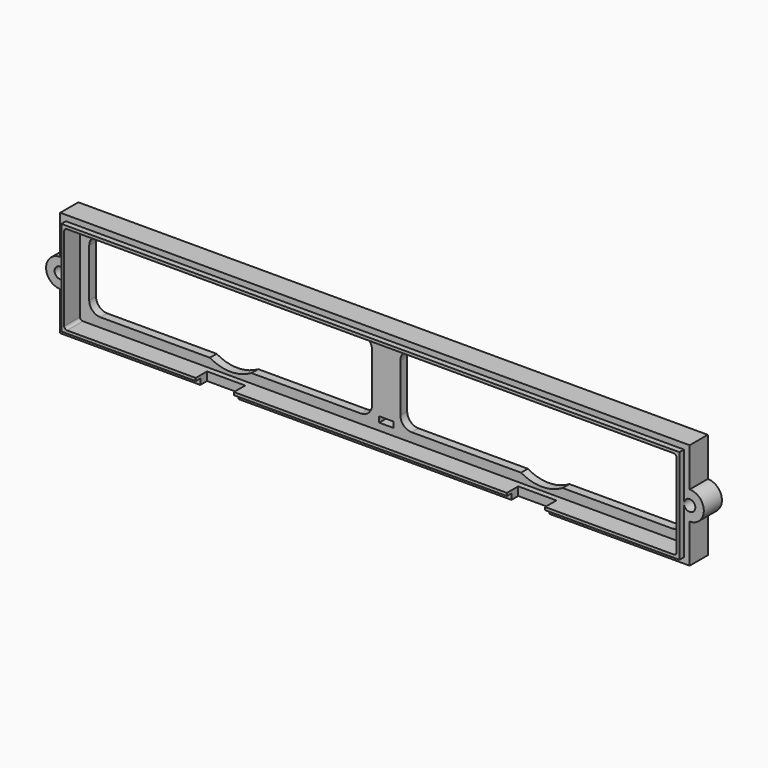
from build123d import *

# Parameters (mm, degrees)
F0_W        = 5
F0_H        = 2
F1_DEPTH    = 3
F2_R        = 2
F3_DEPTH    = 5
F4_W        = 218.5
F4_H        = 33.5
F5_DEPTH    = 2
F6_W        = 13.5
F6_H        = 5
F7_DEPTH    = 25
F8_T1_DEPTH = 5


# Not quite as in the source:
# - a fillet or chamfer that OpenCascade refuses, or shapes differently, is made with other operations: its cross-section is extruded or revolved along the edge and cut away or added
# - a feature names something its author has since deleted; it is built from what else it names


with BuildPart() as f1:
    # F0 (on Front) → F1 (new body)
    with BuildSketch(Plane.XZ):
        Polygon((111.25, 5), (111.25, 18.75), (-111.25, 18.75), (-111.25, 5), (-111.25, -5), (-111.25, -18.75), (111.25, -18.75), (111.25, -5), align=None)
        with Locations((0, -12.25)):
            Rectangle(F0_W, F0_H, mode=Mode.SUBTRACT)
        with BuildLine():
            Line((-47.6515307717, 12.5), (-9, 12.5))
            ThreePointArc((-9, 12.5), (-6.1715728753, 11.3284271247), (-5, 8.5))
            Line((-5, 8.5), (-5, -8.5))
            ThreePointArc((-5, -8.5), (-6.1715728753, -11.3284271247), (-9, -12.5))
            Line((-9, -12.5), (-47.6515307717, -12.5))
            ThreePointArc((-47.6515307717, -12.5), (-55, -14.5), (-62.3484692283, -12.5))
            Line((-62.3484692284, -12.5), (-101, -12.5))
            ThreePointArc((-101, -12.5), (-103.8284271247, -11.3284271247), (-105, -8.5))
            Line((-105, -8.5), (-105, 8.5))
            ThreePointArc((-105, 8.5), (-103.8284271247, 11.3284271247), (-101, 12.5))
            Line((-101, 12.5), (-62.3484692284, 12.5))
            ThreePointArc((-62.3484692283, 12.5), (-55, 14.5), (-47.6515307717, 12.5))
        make_face(mode=Mode.SUBTRACT)
        with BuildLine():
            Line((62.3484692283, 12.5), (101, 12.5))
            ThreePointArc((101, 12.5), (103.8284271247, 11.3284271247), (105, 8.5))
            Line((105, 8.5), (105, -8.5))
            ThreePointArc((105, -8.5), (103.8284271247, -11.3284271247), (101, -12.5))
            Line((101, -12.5), (62.3484692283, -12.5))
            ThreePointArc((62.3484692283, -12.5), (55, -14.5), (47.6515307717, -12.5))
            Line((47.6515307716, -12.5), (9, -12.5))
            ThreePointArc((9, -12.5), (6.1715728753, -11.3284271247), (5, -8.5))
            Line((5, -8.5), (5, 8.5))
            ThreePointArc((5, 8.5), (6.1715728753, 11.3284271247), (9, 12.5))
            Line((9, 12.5), (47.6515307716, 12.5))
            ThreePointArc((47.6515307717, 12.5), (55, 14.5), (62.3484692283, 12.5))
        make_face(mode=Mode.SUBTRACT)
        with Locations((0, 12.25)):
            Rectangle(F0_W, F0_H, mode=Mode.SUBTRACT)
        with BuildLine():
            ThreePointArc((111.25, -5), (116.25, 0), (111.25, 5))
            Line((111.25, 5), (111.25, -5))
        make_face()
        with BuildLine():
            Line((-111.25, -5), (-111.25, 5))
            ThreePointArc((-111.25, 5), (-116.25, 0), (-111.25, -5))
        make_face()
    extrude(amount=F1_DEPTH)

    # F2 (on face) → F3 (join)
    with BuildSketch(Plane.XZ.offset(3)):
        with BuildLine():
            ThreePointArc((111.25, -5), (116.25, 0), (111.25, 5))
            Line((111.25, 5), (111.25, 18.75))
            Line((111.25, 18.75), (-111.25, 18.75))
            Line((-111.25, 18.75), (-111.25, 5))
            ThreePointArc((-111.25, 5), (-116.25, 0), (-111.25, -5))
            Line((-111.25, -5), (-111.25, -18.75))
            Line((-111.25, -18.75), (111.25, -18.75))
            Line((111.25, -18.75), (111.25, -5))
        make_face()
        with Locations((-111.25, 0)):
            Circle(F2_R, mode=Mode.SUBTRACT)
        with BuildLine():
            Line((-107.25, 15.75), (107.25, 15.75))
            ThreePointArc((107.25, 15.75), (107.9571067812, 15.4571067812), (108.25, 14.75))
            Line((108.25, 14.75), (108.25, -14.75))
            ThreePointArc((108.25, -14.75), (107.9571067812, -15.4571067812), (107.25, -15.75))
            Line((107.25, -15.75), (-107.25, -15.75))
            ThreePointArc((-107.25, -15.75), (-107.9571067812, -15.4571067812), (-108.25, -14.75))
            Line((-108.25, -14.75), (-108.25, 14.75))
            ThreePointArc((-108.25, 14.75), (-107.9571067812, 15.4571067812), (-107.25, 15.75))
        make_face(mode=Mode.SUBTRACT)
        with Locations((111.25, 0)):
            Circle(F2_R, mode=Mode.SUBTRACT)
    extrude(amount=F3_DEPTH)

    # F4 (on face) → F5 (join)
    with BuildSketch(Plane.XZ.offset(8)):
        Rectangle(F4_W, F4_H)
        with BuildLine():
            ThreePointArc((-108.25, 14.75), (-107.9571067812, 15.4571067812), (-107.25, 15.75))
            Line((-107.25, 15.75), (107.25, 15.75))
            ThreePointArc((107.25, 15.75), (107.9571067812, 15.4571067812), (108.25, 14.75))
            Line((108.25, 14.75), (108.25, -14.75))
            ThreePointArc((108.25, -14.75), (107.9571067812, -15.4571067812), (107.25, -15.75))
            Line((107.25, -15.75), (-107.25, -15.75))
            ThreePointArc((-107.25, -15.75), (-107.9571067812, -15.4571067812), (-108.25, -14.75))
            Line((-108.25, -14.75), (-108.25, 14.75))
        make_face(mode=Mode.SUBTRACT)
    extrude(amount=F5_DEPTH)

    # F6 (on face) → F7 (cut)
    with BuildSketch(Plane(origin=(0, 0, -18.75), x_dir=(1, 0, 0), z_dir=(0, 0, -1))):
        with Locations((-55, 7.5)):
            Rectangle(F6_W, F6_H)
        with Locations((55, 7.5)):
            Rectangle(F6_W, F6_H)
    extrude(amount=-F7_DEPTH, mode=Mode.SUBTRACT)

    # F8: fillet of radius 3.5 on 2 edges, made by hand

    # F8_s2 → F8_t1 (cut)
    with BuildSketch(Plane.YZ.offset(-2.5)):
        with BuildLine():
            ThreePointArc((0, 7.7858983849), (-0.8542486889, 10.0771862323), (-3, 11.25))
            Line((-3, 11.25), (0, 11.25))
            Line((0, 11.25), (0, 7.7858983849))
        make_face()
        with BuildLine():
            ThreePointArc((0, -7.7858983849), (-0.8542486889, -10.0771862323), (-3, -11.25))
            Line((-3, -11.25), (0, -11.25))
            Line((0, -11.25), (0, -7.7858983849))
        make_face()
    extrude(amount=F8_T1_DEPTH, mode=Mode.SUBTRACT)


solid = f1.part
